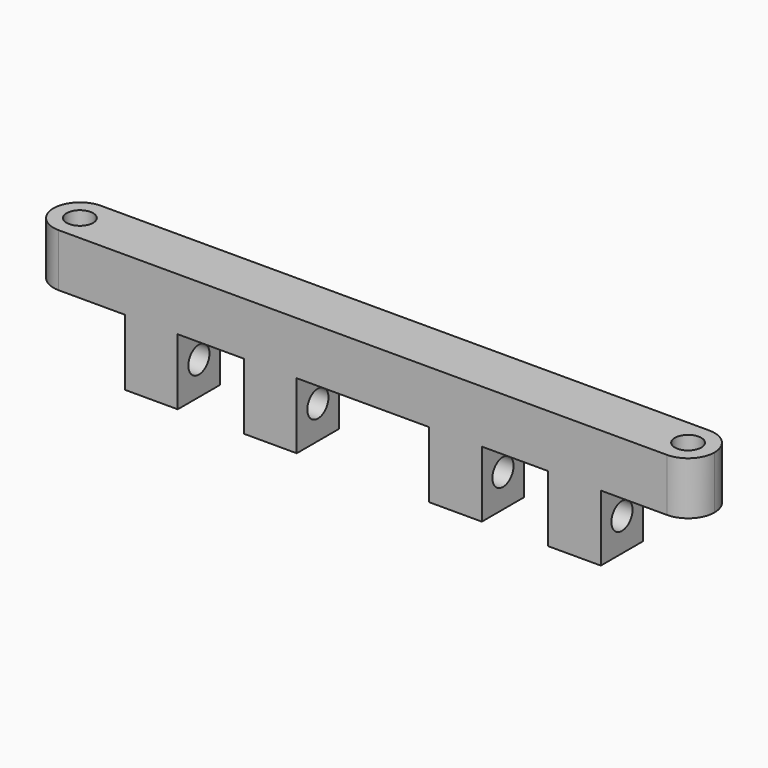
from build123d import *

# Parameters (mm, degrees)
F0_W     = 127
F0_H     = 10.16
F1_DEPTH = 10.16
F2_R     = 5.07999
F3_R     = 2.54
F4_DEPTH = 25.4
F5_W     = 10.16
F5_H     = 10.16
F6_DEPTH = 12.7
F7_R     = 2.54
F8_DEPTH = 99.822


# Not quite as in the source:
# - a fillet or chamfer is up to 0.001 mm smaller than in the source, because OpenCascade refuses the exact size
# - a pattern or mirror of a feature is missing from the dataset's text; its kind, count and spacing are read off the source's solid


with BuildPart() as f1:
    # F0 (on Top) → F1 (new body)
    with BuildSketch(Plane.XY):
        Rectangle(F0_W, F0_H)
    extrude(amount=F1_DEPTH)

    # F2 (radius 5.08 in the source; OpenCascade refuses exactly that, so slightly less here)
    f2_edges = [f1.edges().sort_by_distance(p)[0] for p in [
        (-63.5, -5.08, 5.08),
        (-63.5, 5.08, 5.08),
        (63.5, -5.08, 5.08),
        (63.5, 5.08, 5.08),
    ]]
    fillet(f2_edges, radius=F2_R)

    # F3 (on face) → F4 (cut)
    with BuildSketch(Plane(origin=(0, 0, 0), x_dir=(1, 0, 0), z_dir=(0, 0, -1))):
        with Locations((-58.42, 0)):
            Circle(F3_R)
    f4 = extrude(amount=-F4_DEPTH, mode=Mode.SUBTRACT)

    # F4_copies: F4 across plane
    add(f4.mirror(Plane(origin=(0, 0, 0), x_dir=(0, 0, 1), z_dir=(1, 0, 0))), mode=Mode.SUBTRACT)

    # F5 (on face) → F6 (join)
    with BuildSketch(Plane(origin=(0, 0, 0), x_dir=(1, 0, 0), z_dir=(0, 0, -1))):
        with Locations((-40.64, 0)):
            Rectangle(F5_W, F5_H)
        with Locations((-17.78, 0)):
            Rectangle(F5_W, F5_H)
        with Locations((17.78, 0)):
            Rectangle(F5_W, F5_H)
        with Locations((40.64, 0)):
            Rectangle(F5_W, F5_H)
    extrude(amount=F6_DEPTH)

    # F7 (on face) → F8 (cut)
    with BuildSketch(Plane(origin=(-45.72, 0, 0), x_dir=(0, -1, 0), z_dir=(-1, 0, 0))):
        with Locations((0, -6.35)):
            Circle(F7_R)
    extrude(amount=-F8_DEPTH, mode=Mode.SUBTRACT)


solid = f1.part
